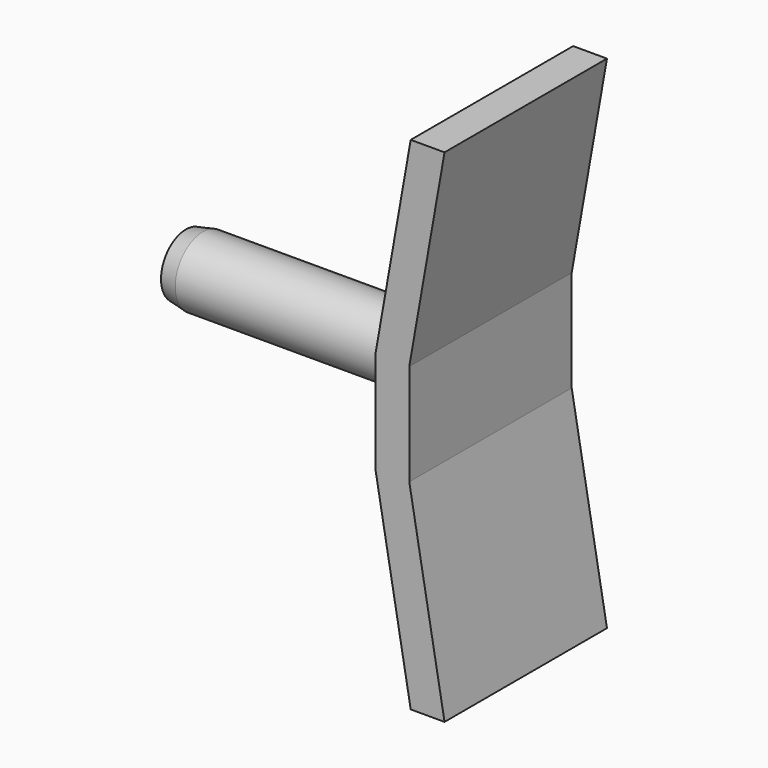
from build123d import *

# Parameters (mm, degrees)
F0_W     = 10
F0_H     = 30
F1_DEPTH = 60
F2_R     = 10.2
F3_DEPTH = 80
F4_SIZE2 = 5
F4_SIZE  = 1


with BuildPart() as f1:
    # F0 (on Front) → F1 (new body)
    with BuildSketch(Plane.XZ):
        Polygon((5.41889066, 74.0884651807), (-5, 15), (5, 15), (15.41889066, 74.0884651807), align=None)
        Rectangle(F0_W, F0_H)
        Polygon((5, -15), (-5, -15), (5.41889066, -74.0884651807), (15.41889066, -74.0884651807), align=None)
    extrude(amount=F1_DEPTH)

    # F2 (on face) → F3 (join)
    with BuildSketch(Plane(origin=(-5, 0, 0), x_dir=(0, -1, 0), z_dir=(-1, 0, 0))):
        with Locations((30, 0)):
            Circle(F2_R)
    extrude(amount=F3_DEPTH)

    # F4
    f4_edges = [f1.edges().sort_by_distance(p)[0] for p in [
        (-85, -19.8, 0),
    ]]
    f4_side = f1.faces().sort_by_distance((-85, -30, 0))[0]
    chamfer(f4_edges, length=F4_SIZE, length2=F4_SIZE2, reference=f4_side)


solid = f1.part
